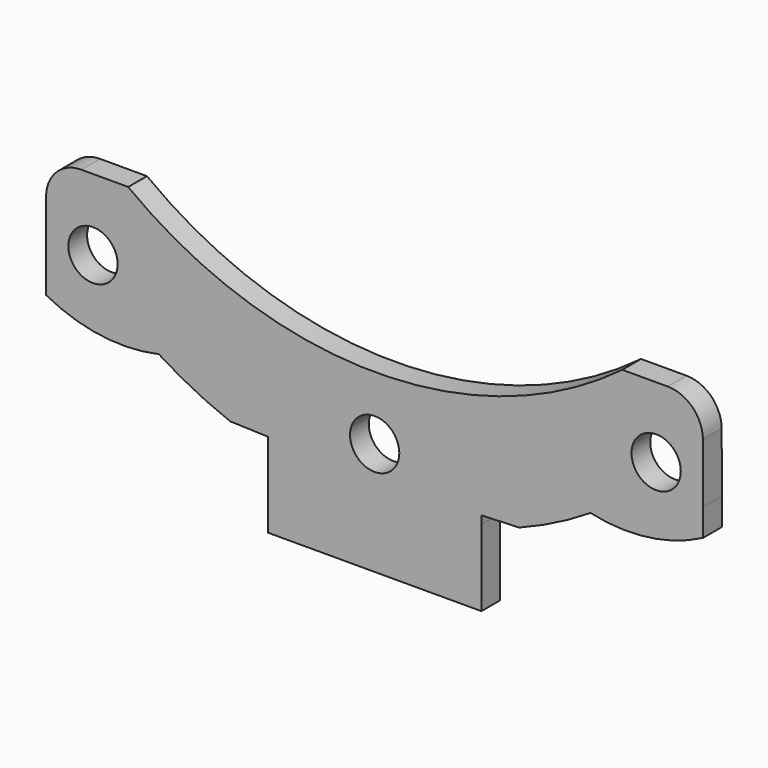
from build123d import *

# Parameters (mm, degrees)
F0_R     = 10.5
F1_DEPTH = 10


# Not quite as in the source:
# - ends of sketch curves that miss each other by under 0.0002 mm in the source are joined


with BuildPart() as f1:
    # F0 (on Front) → F1 (new body)
    with BuildSketch(Plane.XZ):
        with BuildLine():
            Line((-98.7553787733, 42.4647671212), (-118.7477670626, 42.4546280338))
            ThreePointArc((-118.7477670626, 42.4546280338), (-129.3548271656, 38.0531599477), (-133.7401521369, 27.4394155453))
            Line((-133.7401521369, 27.4394155453), (-133.71447629, 2.1254326641))
            Line((-133.71447629, 2.1254326641), (-133.71447629, -9.4965361613))
            ThreePointArc((-133.71447629, -9.4965361613), (-110.2994737436, -17.0606664942), (-85.71447629, -16.0328960194))
            ThreePointArc((-85.71447629, -16.0328960194), (-70.8573251513, -24.4500205619), (-55.2321770125, -31.3375216442))
            Line((-55.2321770125, -31.3375216442), (-39.21447629, -31.8745673359))
            Line((-39.21447629, -31.8745673359), (-39.1571401322, -35.2863552357))
            Line((-39.1571401322, -35.2863552357), (-39.0604409149, -67.8742687524))
            Line((-39.0604409149, -67.8742687524), (51.78552371, -67.7394838983))
            Line((51.78552371, -67.7394838983), (51.78552371, -35.1514269125))
            Line((51.78552371, -35.1514269125), (51.8327357464, -31.7394838983))
            Line((51.8327357464, -31.7394838983), (67.8487723641, -31.1549109155))
            ThreePointArc((67.8487723641, -31.1549109155), (83.4534142883, -24.2210753293), (98.28552371, -15.7599019106))
            ThreePointArc((98.28552371, -15.7599019106), (122.8456433746, -16.920758379), (146.28552371, -9.4965361613))
            Line((146.28552371, -9.4965361613), (146.28552371, 2.1254326641))
            Line((146.28552371, 2.1254326641), (146.1826080128, 27.4394155453))
            ThreePointArc((146.1826080128, 27.4394155453), (141.7598617434, 38.0144245463), (131.1604712744, 42.378416024))
            Line((131.1604712744, 42.378416024), (111.8151785594, 42.3497066713))
            ThreePointArc((111.8151785594, 42.3497066713), (6.5106579482, 7.1928164678), (-98.7553787733, 42.4647671212))
        make_face()
        with Locations((6.2913256733, -19.8069641195)):
            Circle(F0_R, mode=Mode.SUBTRACT)
        with Locations((-113.7560071881, 12.015007423)):
            Circle(F0_R, mode=Mode.SUBTRACT)
        with Locations((126.2437040296, 12.371086267)):
            Circle(F0_R, mode=Mode.SUBTRACT)
    extrude(amount=F1_DEPTH)


solid = f1.part
